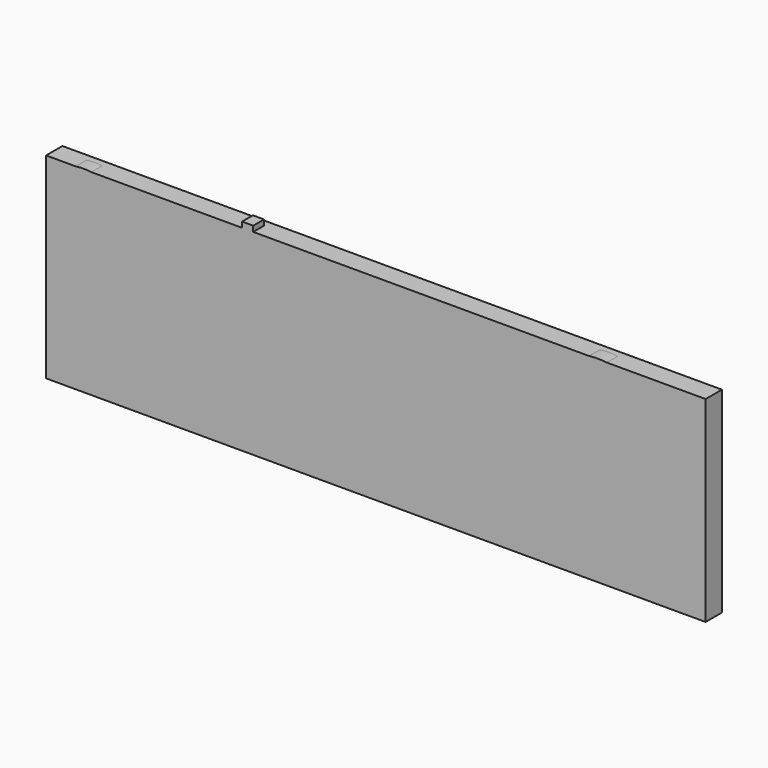
from build123d import *

# Parameters (mm, degrees)
F0_W         = 97
F0_H         = 28.8690390329
F1_DEPTH     = 3
F2_TEXT_SIZE = 20.2149137089
F3_DEPTH     = 2


# Not quite as in the source:
# - Text() gives the source's letters only with a copy of the font that has no kerning and outlines rounded to 1/6400 em; it was checked with that copy


with BuildPart() as f1:
    # F0 (on Front) → F1 (new body)
    with BuildSketch(Plane.XZ):
        with Locations((-6.8255120311, 18.5805219226)):
            Rectangle(F0_W, F0_H)
    extrude(amount=F1_DEPTH)

    # F2 (on face) → F3 (join)
    with BuildSketch(Plane.XZ.offset(3)):
        with Locations((-55.3255120311, 18.4603035686)):
            Text('3rd PLACE', F2_TEXT_SIZE, font='Open Sans', text_align=(TextAlign.LEFT, TextAlign.BOTTOM))
    extrude(amount=-F3_DEPTH)


solid = f1.part
